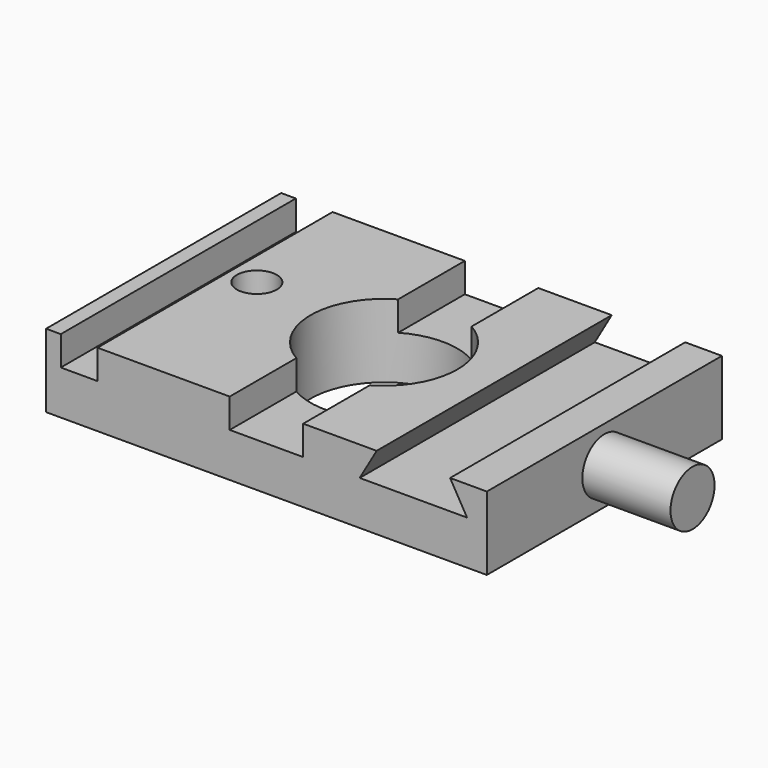
from build123d import *

# Parameters (mm, degrees)
F0_W      = 76.2
F0_H      = 50.8
F0_R      = 12.7
F1_DEPTH  = 12.7
F2_W      = 6.35
F2_H      = 50.8
F3_DEPTH  = 5.08
F5_DEPTH  = 50.801
F6_R      = 4.7625
F7_DEPTH  = 15.24
F8_R      = 3.4489881571
F9_DEPTH  = 12.701
F10_R     = 4.2111787038
F11_DEPTH = 113


# Not quite as in the source:
# - an extrude ends at something that could not be found from the text; its depth is read off the source's solid


with BuildPart() as f1:
    # F0 (on Top) → F1 (new body)
    with BuildSketch(Plane.XY):
        Rectangle(F0_W, F0_H)
        Circle(F0_R, mode=Mode.SUBTRACT)
    extrude(amount=F1_DEPTH)

    # F2 (on face) → F3 (cut)
    with BuildSketch(Plane.XY.offset(12.7)):
        with Locations((-32.385, 0)):
            Rectangle(F2_W, F2_H)
        with BuildLine():
            Line((6.35, 25.4), (-6.35, 25.4))
            Line((-6.35, 25.4), (-6.35, 10.9985226281))
            ThreePointArc((-6.35, 10.9985226281), (0, 12.7), (6.35, 10.9985226281))
            Line((6.35, 10.9985226281), (6.35, 25.4))
        make_face()
        with BuildLine():
            Line((-6.35, -10.9985226281), (-6.35, -25.4))
            Line((-6.35, -25.4), (6.35, -25.4))
            Line((6.35, -25.4), (6.35, -10.9985226281))
            ThreePointArc((6.35, -10.9985226281), (0, -12.7), (-6.35, -10.9985226281))
        make_face()
    extrude(amount=-F3_DEPTH, mode=Mode.SUBTRACT)

    # F4 (on face) → F5 (cut, through all)
    with BuildSketch(Plane.XZ.offset(25.4)):
        Polygon((31.75, 12.7), (19.05, 12.7), (16.1170606325, 7.62), (34.6829393675, 7.62), align=None)
    extrude(amount=-F5_DEPTH, mode=Mode.SUBTRACT)

    # F6 (on face) → F7 (join)
    with BuildSketch(Plane.YZ.offset(38.1)):
        with Locations((0, 6.35)):
            Circle(F6_R)
    extrude(amount=F7_DEPTH)

    # F8 (on face) → F9 (cut, through all)
    with BuildSketch(Plane.XY.offset(12.7)):
        with Locations((-24.371592328, 2.9855815228)):
            Circle(F8_R)
    extrude(amount=-F9_DEPTH, mode=Mode.SUBTRACT)

    # F10 (on face) → F11 (cut, through all)
    with BuildSketch(Plane.XY.offset(12.7)):
        with Locations((-20.9910459816, -11.7274438962)):
            Circle(F10_R)
    extrude(amount=F11_DEPTH, mode=Mode.SUBTRACT)


solid = f1.part
